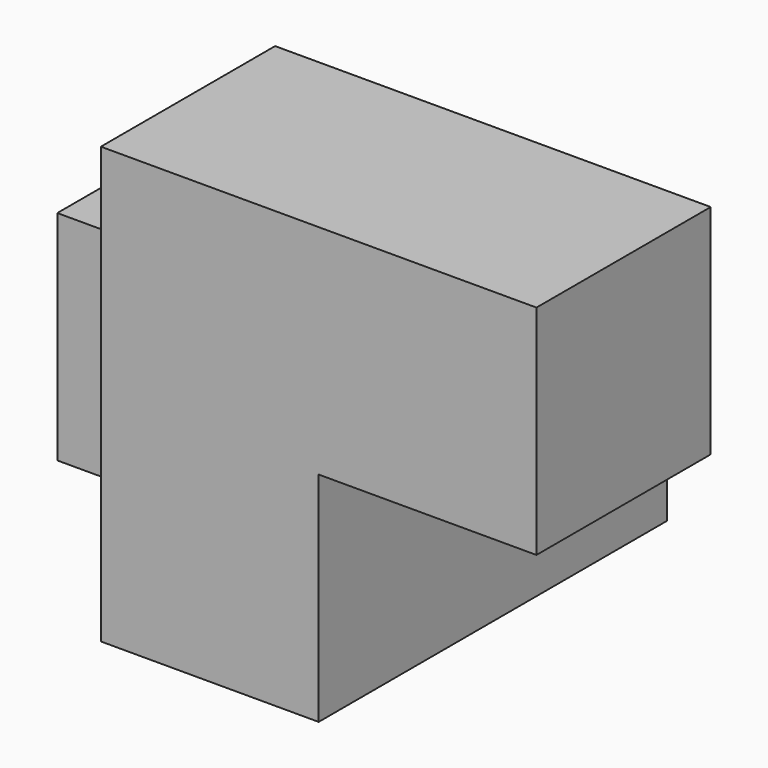
from build123d import *

# Parameters (mm, degrees)
F1_W     = 50.8
F1_H     = 50.8
F2_DEPTH = 50.8
F3_W     = 50.8
F3_H     = 50.8
F4_DEPTH = 50.8
F5_W     = 50.8
F5_H     = 50.8
F6_DEPTH = 101.6
F7_W     = 50.8
F7_H     = 50.8
F8_DEPTH = 50.8


# Not quite as in the source:
# - a variable given as a bare number and used for a length is read in inches; the dataset says mm whatever the document's units were


with BuildPart() as f2:
    # F1 (on Front) → F2 (new body)
    with BuildSketch(Plane.XZ):
        with Locations((3.1213257462, -3.4399425406)):
            Rectangle(F1_W, F1_H)
    extrude(amount=F2_DEPTH)

    # F3 (on face) → F4 (join)
    with BuildSketch(Plane.XZ.offset(50.8)):
        with Locations((53.9213257462, -3.4399425406)):
            Rectangle(F3_W, F3_H)
    extrude(amount=-F4_DEPTH)

    # F5 (on face) → F6 (join)
    with BuildSketch(Plane.XZ.offset(50.8)):
        with Locations((3.1213257462, -54.2399425406)):
            Rectangle(F5_W, F5_H)
    extrude(amount=-F6_DEPTH)

    # F7 (on face) → F8 (join)
    with BuildSketch(Plane(origin=(0, 50.8, 0), x_dir=(-1, 0, 0), z_dir=(0, 1, 0))):
        with Locations((47.6786742538, -54.2399425406)):
            Rectangle(F7_W, F7_H)
    extrude(amount=-F8_DEPTH)


solid = f2.part
